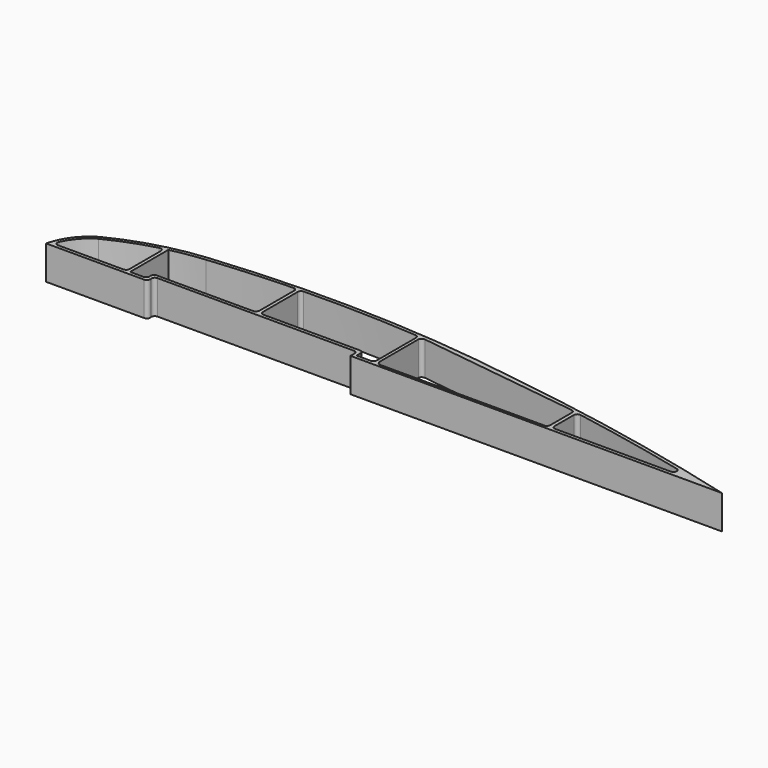
from build123d import *

# Parameters (mm, degrees)
F2_DEPTH = 10
F3_DEPTH = 25


# Not quite as in the source:
# - ends of sketch curves that miss each other by under 0.0002 mm in the source are joined


with BuildPart() as f2:
    # F0 (on Top) → F2 (new body)
    with BuildSketch(Plane.XY):
        with BuildLine():
            ThreePointArc((-442.8758620024, -25.746005996), (-447.6738706777, -30.1036318888), (-450.4042040181, -35.9819879957))
            Line((-450.4042040181, -35.9819879957), (-421.404204, -35.981988))
            ThreePointArc((-421.404204, -35.981988), (-420.6136345975, -35.5943604518), (-420.4359581532, -34.7319880396))
            ThreePointArc((-420.4359581532, -34.7319880396), (-420.2582824791, -33.869615647), (-419.467713, -33.481988))
            Line((-419.467713, -33.481988), (-361.404204, -33.481988))
            ThreePointArc((-361.404204, -33.481988), (-360.6970972188, -33.7748812188), (-360.404204, -34.481988))
            Line((-360.404204, -34.481988), (-360.404204, -35.981988))
            Line((-360.404204, -35.981988), (-250.601554, -35.981988))
            ThreePointArc((-250.601554, -35.981988), (-286.5853141243, -27.5038845491), (-323.0278148887, -21.2867111972))
            ThreePointArc((-323.0278148887, -21.2867111972), (-369.7210642755, -16.7301525977), (-416.6109290422, -18.2670805703))
            ThreePointArc((-416.6109290422, -18.2670805703), (-430.0933310666, -20.7776136638), (-442.8758620024, -25.746005996))
        make_face()
        with BuildLine():
            Line((-428.352885, -34.981988), (-447.624829, -34.981988))
            ThreePointArc((-447.624829, -34.981988), (-448.4629876769, -34.5274144683), (-448.539136854, -33.5769680647))
            ThreePointArc((-448.539136854, -33.5769680647), (-446.0043444552, -29.6253930638), (-442.3948028944, -26.6235058293))
            ThreePointArc((-442.3948028944, -26.6235058293), (-435.6351946925, -23.664150724), (-428.6100890003, -21.4062809989))
            ThreePointArc((-428.6100890003, -21.4062809989), (-427.7434606947, -21.5797937428), (-427.352885, -22.372638))
            Line((-427.352885, -22.372638), (-427.352885, -33.981988))
            ThreePointArc((-427.352885, -33.981988), (-427.6457782188, -34.6890947812), (-428.352885, -34.981988))
        make_face(mode=Mode.SUBTRACT)
        with BuildLine():
            Line((-266.576135, -34.981988), (-300.669352, -34.981988))
            ThreePointArc((-300.669352, -34.981988), (-301.3764587812, -34.6890947812), (-301.669352, -33.981988))
            Line((-301.669352, -33.981988), (-301.669352, -26.854735))
            ThreePointArc((-301.669352, -26.854735), (-301.3113539709, -26.0880320136), (-300.4936850613, -25.8702853433))
            ThreePointArc((-300.4936850613, -25.8702853433), (-283.3655471026, -29.1880608225), (-266.3427238914, -33.0096095475))
            ThreePointArc((-266.3427238914, -33.0096095475), (-265.5830644686, -34.0995078695), (-266.576135, -34.981988))
        make_face(mode=Mode.SUBTRACT)
        with BuildLine():
            Line((-355.237147, -34.981988), (-359.404204, -34.981988))
            Line((-359.404204, -34.981988), (-359.404204, -33.481372))
            ThreePointArc((-359.404204, -33.481372), (-359.6970972188, -32.7742652188), (-360.404204, -32.481372))
            Line((-360.404204, -32.481372), (-388.903588, -32.481372))
            ThreePointArc((-388.903588, -32.481372), (-389.6106947812, -32.1884787812), (-389.903588, -31.481372))
            Line((-389.903588, -31.481372), (-389.903588, -18.621537))
            ThreePointArc((-389.903588, -18.621537), (-389.618081173, -17.9218945872), (-388.9245889886, -17.6217575451))
            ThreePointArc((-388.9245889886, -17.6217575451), (-372.0342144327, -17.6632701711), (-355.1643750064, -18.4969330873))
            ThreePointArc((-355.1643750064, -18.4969330873), (-354.5047632307, -18.8133899275), (-354.237147, -19.494282))
            Line((-354.237147, -19.494282), (-354.237147, -33.981988))
            ThreePointArc((-354.237147, -33.981988), (-354.5300402188, -34.6890947812), (-355.237147, -34.981988))
        make_face(mode=Mode.SUBTRACT)
    extrude(amount=F2_DEPTH)

    # F1 (on face) → F3 (cut)
    with BuildSketch(Plane.XY):
        with BuildLine():
            Line((-426.3566434383, -20.8794865757), (-426.3566434383, -34.9726714194))
            Line((-426.3566434383, -34.9726714194), (-422.3857820034, -34.994803369))
            ThreePointArc((-422.3857820034, -34.994803369), (-421.6962703088, -34.6752877171), (-421.401143074, -33.9749902487))
            Line((-421.401143074, -33.9749902487), (-421.4363098145, -33.4650874138))
            ThreePointArc((-421.4363098145, -33.4650874138), (-421.0609978365, -32.7289703218), (-420.2582538128, -32.5331911445))
            Line((-420.2582538128, -32.5331911445), (-391.879349947, -32.5331911445))
            ThreePointArc((-391.879349947, -32.5331911445), (-391.1928137109, -32.1470446257), (-390.9206390381, -31.4078815281))
            Line((-390.9206390381, -31.4078815281), (-390.9206390381, -18.7257640064))
            ThreePointArc((-390.9206390381, -18.7257640064), (-391.1852808069, -17.9443289757), (-391.9595777988, -17.6594778895))
            ThreePointArc((-391.9595777988, -17.6594778895), (-404.2164737194, -18.2651978438), (-416.4454340935, -19.290342927))
            ThreePointArc((-416.4454340935, -19.290342927), (-421.4266657547, -19.925083731), (-426.3566434383, -20.8794865757))
        make_face()
        with BuildLine():
            Line((-353.3217906952, -19.678786397), (-353.3217906952, -33.9749902487))
            ThreePointArc((-353.3217906952, -33.9749902487), (-353.0459602673, -34.7694772845), (-352.3371517658, -35.2221168578))
            Line((-352.3371517658, -35.2221168578), (-303.7378787994, -35.2221168578))
            ThreePointArc((-303.7378787994, -35.2221168578), (-302.935974646, -34.8299169031), (-302.7532398701, -33.9561440051))
            Line((-302.7532398701, -33.9561440051), (-302.7532398701, -26.2196455151))
            ThreePointArc((-302.7532398701, -26.2196455151), (-302.9931053965, -25.5712210446), (-303.5972118378, -25.2349991351))
            Line((-303.5972118378, -25.2349991351), (-352.1261513233, -18.8348051161))
            ThreePointArc((-352.1261513233, -18.8348051161), (-352.8890528033, -19.0229300334), (-353.3217906952, -19.678786397))
        make_face()
    extrude(amount=F3_DEPTH, mode=Mode.SUBTRACT)


solid = f2.part
